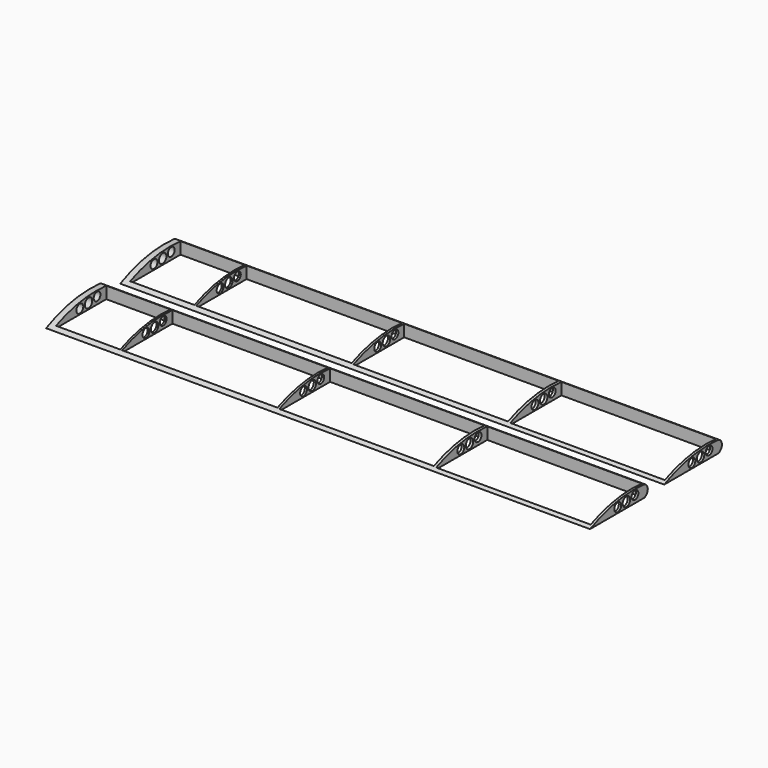
from build123d import *

# Parameters (mm, degrees)
F1_DEPTH  = 360.68
F2_R      = 3.2120492673
F3_DEPTH  = 63.754
F5_R      = 2.8036172984
F6_DEPTH  = 762
F7_R      = 3.0895845535
F8_DEPTH  = 780.796
F9_R      = 2.8613866687
F10_DEPTH = 1653.54
F12_W     = 102.4557352066
F12_H     = 42.3665232956
F13_DEPTH = 404.114
F14_W     = 102.4557352066
F14_H     = 42.0261770487
F15_DEPTH = 473.202
F16_W     = 103.0241213739
F16_H     = 41.7147055268
F17_DEPTH = 452.374
F18_W     = 42.6017828286
F18_H     = 41.6653864086
F19_DEPTH = 565.404


# Not quite as in the source:
# - a feature names something its author has since deleted; it is built from what else it names


with BuildPart() as f1:
    # F0 (on Right) → F1 (new body)
    with BuildSketch(Plane.YZ):
        with BuildLine():
            Line((-44.8486544192, 0), (0, 0))
            ThreePointArc((0, 0), (2.991656056, 3.9466815069), (0, 7.8933630139))
            ThreePointArc((0, 7.8933630139), (-22.9601802311, 6.9913010105), (-44.8486544192, 0))
        make_face()
    extrude(amount=F1_DEPTH)

    # F2 (on face) → F3 (cut)
    with BuildSketch(Plane.YZ.offset(360.68)):
        with Locations((-1.1074616928, 3.9466815069)):
            Circle(F2_R)
    extrude(amount=F3_DEPTH, mode=Mode.SUBTRACT)

    # F5 (on offset) → F6 (cut)
    with BuildSketch(Plane.YZ.offset(728.98)):
        with Locations((-7.6232864521, 4.759835545)):
            Circle(F5_R)
    extrude(amount=-F6_DEPTH, mode=Mode.SUBTRACT)

    # F7 (on offset) → F8 (cut)
    with BuildSketch(Plane.YZ.offset(728.98)):
        with Locations((-14.7137921304, 3.8258279674)):
            Circle(F7_R)
    extrude(amount=-F8_DEPTH, mode=Mode.SUBTRACT)

    # F9 (on offset) → F10 (cut)
    with BuildSketch(Plane.YZ.offset(728.98)):
        with Locations((-21.9230763614, 3.4620482475)):
            Circle(F9_R)
    extrude(amount=-F10_DEPTH, mode=Mode.SUBTRACT)

    # F12 (on offset) → F13 (cut)
    with BuildSketch(Plane.XY.offset(-200.66)):
        with Locations((307.8756928444, -21.1832616478)):
            Rectangle(F12_W, F12_H)
    extrude(amount=F13_DEPTH, mode=Mode.SUBTRACT)

    # F14 (on offset) → F15 (cut)
    with BuildSketch(Plane.XY.offset(-200.66)):
        with Locations((203.6147117615, -21.0130885243)):
            Rectangle(F14_W, F14_H)
    extrude(amount=F15_DEPTH, mode=Mode.SUBTRACT)

    # F16 (on offset) → F17 (cut)
    with BuildSketch(Plane.XY.offset(-200.66)):
        with Locations((99.4069892913, -20.8573527634)):
            Rectangle(F16_W, F16_H)
    extrude(amount=F17_DEPTH, mode=Mode.SUBTRACT)

    # F18 (on offset) → F19 (cut)
    with BuildSketch(Plane.XY.offset(-200.66)):
        with Locations((25.3316406161, -20.8326932043)):
            Rectangle(F18_W, F18_H)
    extrude(amount=F19_DEPTH, mode=Mode.SUBTRACT)


with BuildPart() as f20_1:
    # F20: copy of F1
    add(f1.part.moved(Location((0, 61.468, 1.016))))


solid = Compound([f1.part, f20_1.part])
